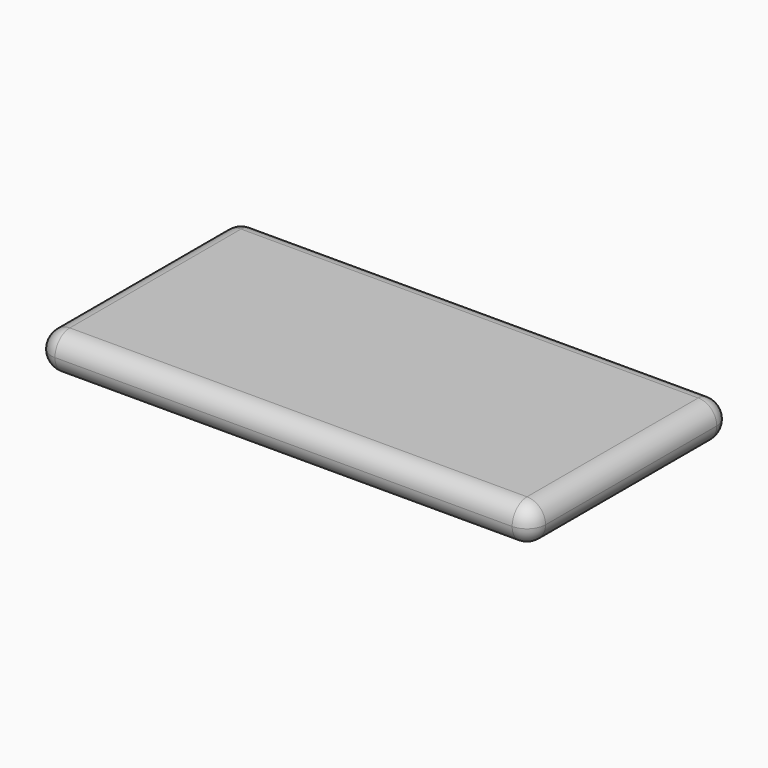
from build123d import *

# Parameters (mm, degrees)
F0_W     = 133.2894712687
F0_H     = 67.712135613
F1_DEPTH = 10
F2_R     = 4.99999
F3_T     = -2.5


# Not quite as in the source:
# - a fillet or chamfer is up to 0.001 mm smaller than in the source, because OpenCascade refuses the exact size


with BuildPart() as f1:
    # F0 (on Top) → F1 (new body)
    with BuildSketch(Plane.XY):
        Rectangle(F0_W, F0_H)
    extrude(amount=F1_DEPTH)

    # F2 (radius 5 in the source; OpenCascade refuses exactly that, so slightly less here)
    f2_edges = [f1.edges().sort_by_distance(p)[0] for p in [
        (66.644736, 33.856068, 5),
        (-66.644736, 33.856068, 5),
        (0, 33.856068, 0),
        (0, 33.856068, 10),
        (-66.644736, -33.856068, 5),
        (-66.644736, 0, 0),
        (-66.644736, 0, 10),
        (66.644736, -33.856068, 5),
        (0, -33.856068, 0),
        (0, -33.856068, 10),
        (66.644736, 0, 0),
        (66.644736, 0, 10),
    ]]
    fillet(f2_edges, radius=F2_R)

    # F3 (hollow: no face is removed)
    offset(amount=F3_T, mode=Mode.SUBTRACT)


solid = f1.part
